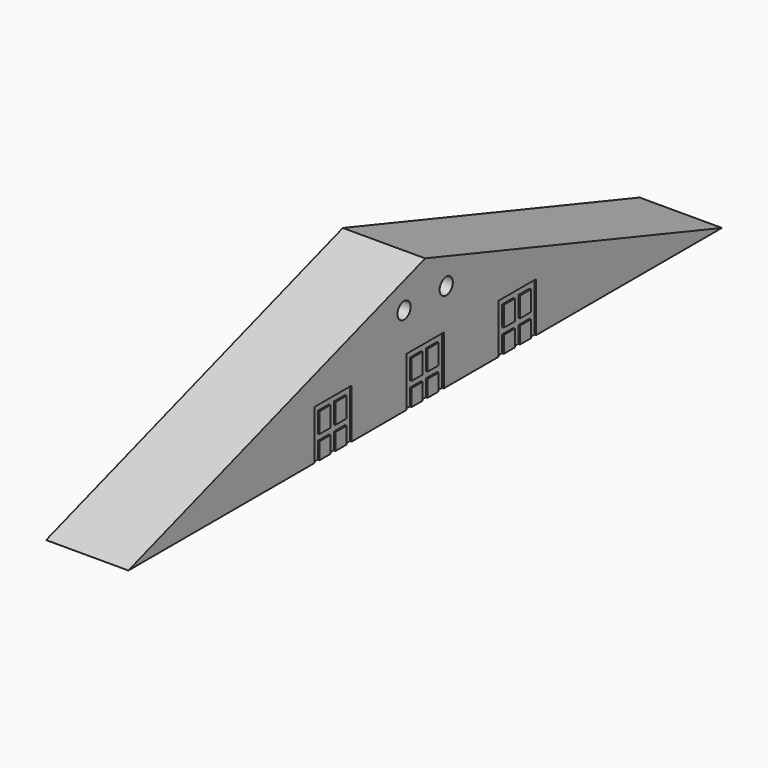
from build123d import *

# Parameters (mm, degrees)
F1_DEPTH  = 8
F3_DEPTH  = 621.7
F4_DEPTH  = 5.5
F7_DEPTH  = 5.5
F9_DEPTH  = 5.5
F11_DEPTH = 5.5
F13_DEPTH = 5.5
F15_DEPTH = 5.5
F17_DEPTH = 308.2
F18_DEPTH = 24
F20_DEPTH = 244.2
F21_DEPTH = 30.35
F22_R     = 2.5
F23_DEPTH = 0.5
F24_R     = 2.5
F25_DEPTH = 0.5
F26_R     = 2.5
F27_DEPTH = 0.5
F28_R     = 2.5
F29_DEPTH = 0.5
F30_W     = 14.1428571429
F30_H     = 18
F30_W_2   = 4.1785714286
F30_H_2   = 6.1071428571
F31_DEPTH = 0.5
F32_DEPTH = 25
F34_DEPTH = 8
F35_DEPTH = 0.5
F36_W     = 4.1785714286
F36_H     = 6.1071428571
F36_H_2   = 5.0357142857
F37_DEPTH = 24.5
F38_DEPTH = 25
F39_DEPTH = 1.05


# Not quite as in the source:
# - a feature of the source that left no trace in its solid (it failed there, or was rolled back) is left out


with BuildPart() as f1:
    # F0 (on Top) → F1 (new body)
    with BuildSketch(Plane.XY):
        Polygon((-327.3, 108.1424002851), (-327.3, -140.8575997149), (-102.6, -140.8575997149), (-102.6, -170.8575997149), (0, -170.8575997149), (0, -140.8575997149), (288.9, -140.8575997149), (288.9, 108.1424002851), (0, 108.1424002851), (0, 138.1424002851), (-102.6, 128.6424002851), (-102.6, 108.1424002851), align=None)
    extrude(amount=F1_DEPTH)

    # F2 (on face) → F3 (join)
    with BuildSketch(Plane.YZ.offset(288.9)):
        Polygon((-16.3575997149, 51.4532495908), (-146.3575997149, 8), (-140.8575997149, 8), (108.1424002851, 8), (113.6424002851, 8), align=None)
    extrude(amount=-F3_DEPTH)

    # F2 (on face) → F4 (join)
    with BuildSketch(Plane.YZ.offset(288.9)):
        Polygon((-16.3575997149, 51.4532495908), (-146.3575997149, 8), (113.6424002851, 8), align=None)
    extrude(amount=F4_DEPTH)

    # F5 (on face) → F7 (join)
    with BuildSketch(Plane.XZ.offset(170.8575997149)):
        Polygon((-51.3, 62.75), (-108.1, 8), (5.5, 8), align=None)
    extrude(amount=F7_DEPTH)

    # F8 (on face) → F9 (cut)
    with BuildSketch(Plane(origin=(-13.187163576, 142.4213666207, 0), x_dir=(-0.9957406741, -0.0921982106, 0), z_dir=(-0.0921982106, 0.9957406741, 0))):
        Polygon((91.8565413643, 4.3927081219), (38.2758658123, 55.8195932448), (-15.3048097397, 4.3927081219), align=None)
    extrude(amount=-F9_DEPTH, mode=Mode.SUBTRACT)

    # F10 (on face) → F11 (cut)
    with BuildSketch(Plane(origin=(-332.8, 0, 0), x_dir=(0, -1, 0), z_dir=(-1, 0, 0))):
        Polygon((144.6140170728, 2.7836871671), (16.3575997149, 45.6541342062), (-111.8988176431, 2.7836871671), align=None)
    extrude(amount=-F11_DEPTH, mode=Mode.SUBTRACT)

    # F12 (on face) → F13 (cut)
    with BuildSketch(Plane.YZ.offset(294.4)):
        Polygon((111.8988176431, 2.7836871671), (-16.3575997149, 45.6541342062), (-144.6140170728, 2.7836871671), align=None)
    extrude(amount=-F13_DEPTH, mode=Mode.SUBTRACT)

    # F14 (on face) → F15 (cut)
    with BuildSketch(Plane.XZ.offset(176.3575997149)):
        Polygon((1.6830285492, 4.0401099834), (-51.3, 55.1108989459), (-104.2830285492, 4.0401099834), align=None)
    extrude(amount=-F15_DEPTH, mode=Mode.SUBTRACT)

    # F16 (on face) → F17 (join)
    with BuildSketch(Plane.YZ.offset(294.4)):
        Polygon((-37.9123742622, 48.4659791319), (-36.6443145321, 44.6722981882), (-16.3575997149, 51.4532495908), (3.9291151024, 44.6722981882), (5.1971748325, 48.4659791319), (-16.3575997149, 55.670786811), align=None)
    extrude(amount=-F17_DEPTH)

    # F16 (on face) → F18 (cut)
    with BuildSketch(Plane.YZ.offset(294.4)):
        Polygon((-37.9123742622, 48.4659791319), (-36.6443145321, 44.6722981882), (-16.3575997149, 51.4532495908), (3.9291151024, 44.6722981882), (5.1971748325, 48.4659791319), (-16.3575997149, 55.670786811), align=None)
    extrude(amount=-F18_DEPTH, mode=Mode.SUBTRACT)

    # F19 (on face) → F20 (join)
    with BuildSketch(Plane(origin=(-332.8, 0, 0), x_dir=(0, -1, 0), z_dir=(-1, 0, 0))):
        Polygon((-5.1971748325, 48.4659791319), (-3.9291151024, 44.6722981882), (16.3575997149, 51.4532495908), (36.6443145321, 44.6722981882), (37.9123742622, 48.4659791319), (16.3575997149, 55.670786811), align=None)
    extrude(amount=-F20_DEPTH)

    # F19 (on face) → F21 (cut)
    with BuildSketch(Plane(origin=(-332.8, 0, 0), x_dir=(0, -1, 0), z_dir=(-1, 0, 0))):
        Polygon((-5.1971748325, 48.4659791319), (-3.9291151024, 44.6722981882), (16.3575997149, 51.4532495908), (36.6443145321, 44.6722981882), (37.9123742622, 48.4659791319), (16.3575997149, 55.670786811), align=None)
    extrude(amount=-F21_DEPTH, mode=Mode.SUBTRACT)

    # F22 (on face) → F23 (cut)
    with BuildSketch(Plane(origin=(-327.3, 0, 0), x_dir=(0, -1, 0), z_dir=(-1, 0, 0))):
        with Locations((8.3575997149, 35)):
            Circle(F22_R)
        with Locations((24.3575997149, 35)):
            Circle(F22_R)
    extrude(amount=-F23_DEPTH, mode=Mode.SUBTRACT)

    # F24 (on face) → F25 (cut)
    with BuildSketch(Plane.YZ.offset(288.9)):
        with Locations((-24.3575997149, 35)):
            Circle(F24_R)
        with Locations((-8.3575997149, 35)):
            Circle(F24_R)
    extrude(amount=-F25_DEPTH, mode=Mode.SUBTRACT)

    # F26 (on face) → F27 (cut)
    with BuildSketch(Plane.XZ.offset(170.8575997149)):
        with Locations((-59.3, 35)):
            Circle(F26_R)
        with Locations((-43.3, 35)):
            Circle(F26_R)
    extrude(amount=-F27_DEPTH, mode=Mode.SUBTRACT)

    # F28 (on face) → F29 (cut)
    with BuildSketch(Plane(origin=(-12.6822332802, 136.9681194259, 0), x_dir=(-0.9957406741, -0.0921982106, 0), z_dir=(-0.0921982106, 0.9957406741, 0))):
        with Locations((30.7829559704, 35)):
            Circle(F28_R)
        with Locations((46.7829559704, 35)):
            Circle(F28_R)
    extrude(amount=-F29_DEPTH, mode=Mode.SUBTRACT)

    # F30 (on face) → F31 (cut)
    with BuildSketch(Plane.YZ.offset(288.9)):
        with Locations((-16.3575997149, 14)):
            Rectangle(F30_W, F30_H)
        with Locations((-19.4111711434, 9.9821428571)):
            Rectangle(F30_W_2, F30_H_2, mode=Mode.SUBTRACT)
        with Locations((-13.3040282863, 9.9821428571)):
            Rectangle(F30_W_2, F30_H_2, mode=Mode.SUBTRACT)
        with Locations((-19.4111711434, 18.0178571429)):
            Rectangle(F30_W_2, F30_H_2, mode=Mode.SUBTRACT)
        with Locations((-13.3040282863, 18.0178571429)):
            Rectangle(F30_W_2, F30_H_2, mode=Mode.SUBTRACT)
        with Locations((18.6424002851, 14)):
            Rectangle(F30_W, F30_H)
        with Locations((15.5888288566, 9.9821428571)):
            Rectangle(F30_W_2, F30_H_2, mode=Mode.SUBTRACT)
        with Locations((21.6959717137, 9.9821428571)):
            Rectangle(F30_W_2, F30_H_2, mode=Mode.SUBTRACT)
        with Locations((15.5888288566, 18.0178571429)):
            Rectangle(F30_W_2, F30_H_2, mode=Mode.SUBTRACT)
        with Locations((21.6959717137, 18.0178571429)):
            Rectangle(F30_W_2, F30_H_2, mode=Mode.SUBTRACT)
        with Locations((-51.3575997149, 14)):
            Rectangle(F30_W, F30_H)
        with Locations((-54.4111711434, 9.9821428571)):
            Rectangle(F30_W_2, F30_H_2, mode=Mode.SUBTRACT)
        with Locations((-48.3040282863, 9.9821428571)):
            Rectangle(F30_W_2, F30_H_2, mode=Mode.SUBTRACT)
        with Locations((-54.4111711434, 18.0178571429)):
            Rectangle(F30_W_2, F30_H_2, mode=Mode.SUBTRACT)
        with Locations((-48.3040282863, 18.0178571429)):
            Rectangle(F30_W_2, F30_H_2, mode=Mode.SUBTRACT)
    extrude(amount=-F31_DEPTH, mode=Mode.SUBTRACT)


with BuildPart() as f32:
    # F32 (new): faces of the model
    f32_faces = [f1.part.faces().sort_by_distance(p)[0] for p in [
        (288.9, -16.3575997149, 2.5315074555),
        (288.4, -51.3575997149, 14),
        (288.4, -16.3575997149, 14),
        (288.4, 18.6424002851, 14),
    ]]
    extrude(f32_faces, amount=F32_DEPTH)

    # F34 (cut): a face of the model
    f34_faces = [f32.faces().sort_by_distance(p)[0] for p in [
        (301.4, -16.3575997149, 0),
    ]]
    extrude(f34_faces, amount=-F34_DEPTH, mode=Mode.SUBTRACT)

    # F35 (cut): faces of the model
    f35_faces = [f32.faces().sort_by_distance(p)[0] for p in [
        (288.4, 18.6424002851, 14),
        (288.4, -16.3575997149, 14),
        (288.4, -51.3575997149, 14),
    ]]
    extrude(f35_faces, amount=-F35_DEPTH, mode=Mode.SUBTRACT)

    # F36 (on face) → F37 (join)
    with BuildSketch(Plane(origin=(288.9, 0, 0), x_dir=(0, -1, 0), z_dir=(-1, 0, 0))):
        Polygon((61.9918890297, 25.6764385849), (-32.9998731613, 25.6764385849), (-32.9998731613, 8), (-23.785257428, 8), (-23.785257428, 13.0357142857), (-19.6066859994, 13.0357142857), (-19.6066859994, 8), (-17.6781145709, 8), (-17.6781145709, 13.0357142857), (-13.4995431423, 13.0357142857), (-13.4995431423, 8), (11.214742572, 8), (11.214742572, 13.0357142857), (15.3933140006, 13.0357142857), (15.3933140006, 8), (17.3218854291, 8), (17.3218854291, 13.0357142857), (21.5004568577, 13.0357142857), (21.5004568577, 8), (46.214742572, 8), (46.214742572, 13.0357142857), (50.3933140006, 13.0357142857), (50.3933140006, 8), (52.3218854291, 8), (52.3218854291, 13.0357142857), (56.5004568577, 13.0357142857), (56.5004568577, 8), (61.9918890297, 8), align=None)
        with Locations((-21.6959717137, 18.0178571429)):
            Rectangle(F36_W, F36_H, mode=Mode.SUBTRACT)
        with Locations((-15.5888288566, 18.0178571429)):
            Rectangle(F36_W, F36_H, mode=Mode.SUBTRACT)
        with Locations((13.3040282863, 18.0178571429)):
            Rectangle(F36_W, F36_H, mode=Mode.SUBTRACT)
        with Locations((19.4111711434, 18.0178571429)):
            Rectangle(F36_W, F36_H, mode=Mode.SUBTRACT)
        with Locations((48.3040282863, 18.0178571429)):
            Rectangle(F36_W, F36_H, mode=Mode.SUBTRACT)
        with Locations((54.4111711434, 18.0178571429)):
            Rectangle(F36_W, F36_H, mode=Mode.SUBTRACT)
        with Locations((-21.6959717137, 18.0178571429)):
            Rectangle(F36_W, F36_H)
        with Locations((-15.5888288566, 18.0178571429)):
            Rectangle(F36_W, F36_H)
        with Locations((-15.5888288566, 10.5178571429)):
            Rectangle(F36_W, F36_H_2)
        with Locations((-21.6959717137, 10.5178571429)):
            Rectangle(F36_W, F36_H_2)
        with Locations((13.3040282863, 18.0178571429)):
            Rectangle(F36_W, F36_H)
        with Locations((19.4111711434, 18.0178571429)):
            Rectangle(F36_W, F36_H)
        with Locations((19.4111711434, 10.5178571429)):
            Rectangle(F36_W, F36_H_2)
        with Locations((13.3040282863, 10.5178571429)):
            Rectangle(F36_W, F36_H_2)
        with Locations((48.3040282863, 18.0178571429)):
            Rectangle(F36_W, F36_H)
        with Locations((54.4111711434, 18.0178571429)):
            Rectangle(F36_W, F36_H)
        with Locations((54.4111711434, 10.5178571429)):
            Rectangle(F36_W, F36_H_2)
        with Locations((48.3040282863, 10.5178571429)):
            Rectangle(F36_W, F36_H_2)
    extrude(amount=-F37_DEPTH)

    # F30 (on face) → F38 (join)
    with BuildSketch(Plane.YZ.offset(288.9)):
        with Locations((21.6959717137, 18.0178571429)):
            Rectangle(F30_W_2, F30_H_2)
        with Locations((15.5888288566, 18.0178571429)):
            Rectangle(F30_W_2, F30_H_2)
        with Locations((15.5888288566, 9.9821428571)):
            Rectangle(F30_W_2, F30_H_2)
        with Locations((21.6959717137, 9.9821428571)):
            Rectangle(F30_W_2, F30_H_2)
        with Locations((-13.3040282863, 18.0178571429)):
            Rectangle(F30_W_2, F30_H_2)
        with Locations((-13.3040282863, 9.9821428571)):
            Rectangle(F30_W_2, F30_H_2)
        with Locations((-19.4111711434, 9.9821428571)):
            Rectangle(F30_W_2, F30_H_2)
        with Locations((-19.4111711434, 18.0178571429)):
            Rectangle(F30_W_2, F30_H_2)
        with Locations((-48.3040282863, 18.0178571429)):
            Rectangle(F30_W_2, F30_H_2)
        with Locations((-54.4111711434, 18.0178571429)):
            Rectangle(F30_W_2, F30_H_2)
        with Locations((-54.4111711434, 9.9821428571)):
            Rectangle(F30_W_2, F30_H_2)
        with Locations((-48.3040282863, 9.9821428571)):
            Rectangle(F30_W_2, F30_H_2)
    extrude(amount=F38_DEPTH)

    # F39 (cut): faces of the model
    f39_faces = [f32.faces().sort_by_distance(p)[0] for p in [
        (301.4, -54.4111711434, 6.9285714286),
        (301.4, -48.3040282863, 6.9285714286),
        (301.4, -19.4111711434, 6.9285714286),
        (301.4, -13.3040282863, 6.9285714286),
        (301.4, 15.5888288566, 6.9285714286),
        (301.4, 21.6959717137, 6.9285714286),
    ]]
    extrude(f39_faces, amount=-F39_DEPTH, mode=Mode.SUBTRACT)


solid = f32.part
